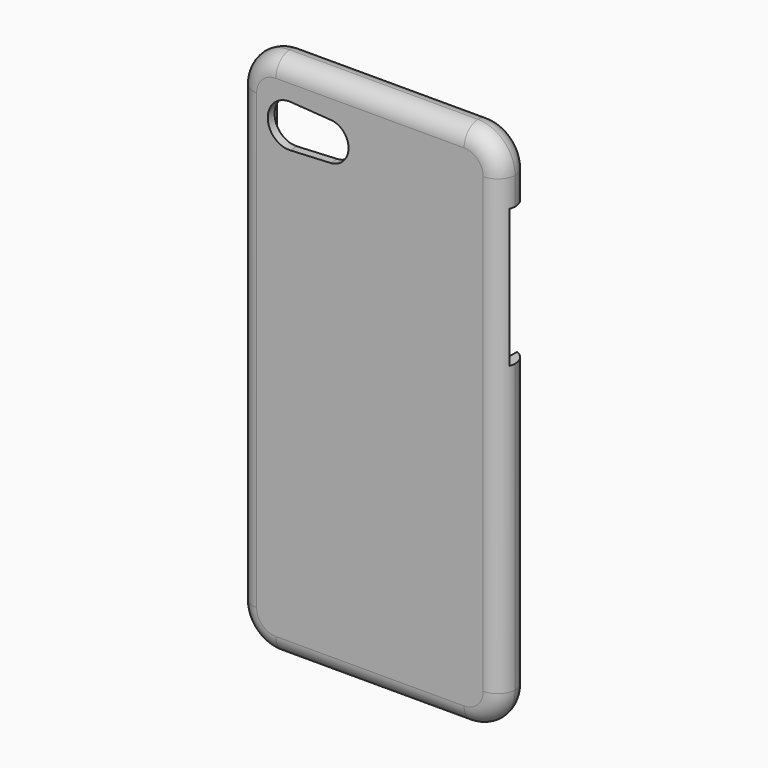
from build123d import *

# Parameters (mm, degrees)
F1_DEPTH      = 9.8298
F2_R          = 10.414
F4_DEPTH      = 7.4422
F6_R          = 10.414
F7_DEPTH      = 25.4
F8_T1_DEPTH   = 126.492
F8_T3_DEPTH   = 52.578
F8_T6_ANGLE   = 90
F8_T8_ANGLE   = 90
F8_T10_ANGLE  = 90
F8_T12_ANGLE  = 90
F9_T1_DEPTH   = 126.492
F9_T3_DEPTH   = 52.578
F9_T6_ANGLE   = 90
F9_T8_ANGLE   = 90
F9_T10_ANGLE  = 90
F9_T12_ANGLE  = 90
F10_W         = 13.4874
F10_H         = 2.8194
F11_DEPTH     = 76.2
F12_W         = 6.6548
F12_H         = 38.608
F13_DEPTH     = 36.7040001
F14_W         = 6.6548
F14_H         = 12.6361389041
F15_DEPTH     = 36.7040001
F16_T1_DEPTH  = 46.228
F16_T6_DEPTH  = 117.348
F16_T11_DEPTH = 117.348
F16_T16_DEPTH = 117.348
F16_T21_ANGLE = 90
F16_T26_ANGLE = 90
F16_T31_ANGLE = 90
F16_T36_ANGLE = 90
F16_T41_DEPTH = 117.348
F16_T46_DEPTH = 117.348
F16_T51_DEPTH = 117.348
F16_T54_ANGLE = 90
F16_T56_ANGLE = 90
F16_T60_DEPTH = 46.228
F16_T66_DEPTH = 46.228
F16_T72_DEPTH = 46.228
F16_T78_DEPTH = 46.228
F16_T83_DEPTH = 46.228


# Not quite as in the source:
# - a fillet or chamfer that OpenCascade refuses, or shapes differently, is made with other operations: its cross-section is extruded or revolved along the edge and cut away or added


with BuildPart() as f1:
    # F0 (on Front) → F1 (new body)
    with BuildSketch(Plane.XZ):
        Polygon((-36.703, -73.66), (36.703, -73.66), (36.703, 73.66), (-26.8460772932, 73.66), (-36.703, 73.66), (-36.703, 59.1852668802), align=None)
        with BuildLine():
            ThreePointArc((-22.2717920435, 52.197646321), (-28.0758079345, 55.8760032584), (-26.5712787061, 62.5807256257))
            ThreePointArc((-26.5712787061, 62.5807256257), (-24.5177487597, 63.7987699714), (-22.1511274544, 64.1145560806))
            Line((-22.1511274544, 64.1145560806), (-10.919338154, 63.3416271462))
            ThreePointArc((-10.919338154, 63.3416271462), (-7.4032650854, 61.6681227759), (-5.9751011246, 58.0454532626))
            ThreePointArc((-5.9751011246, 58.0454532626), (-7.4401434327, 54.3836791207), (-11.0266546305, 52.7429852861))
            Line((-11.0266546305, 52.7429852861), (-22.2717920435, 52.197646321))
        make_face(mode=Mode.SUBTRACT)
    extrude(amount=F1_DEPTH)

    # F2
    f2_edges = [f1.edges().sort_by_distance(p)[0] for p in [
        (36.703, -4.9149, -73.66),
        (36.703, -4.9149, 73.66),
        (-36.703, -4.9149, -73.66),
        (-36.703, -4.9149, 73.66),
    ]]
    fillet(f2_edges, radius=F2_R)

    # F3 (on Front) → F4 (cut)
    with BuildSketch(Plane.XZ):
        Polygon((-33.528, -69.088), (33.528, -69.088), (33.528, 69.088), (-6.3646039926, 69.088), (-33.528, 69.088), (-33.528, -30.0187896937), align=None)
    extrude(amount=F4_DEPTH, mode=Mode.SUBTRACT)

    # F6
    f6_edges = [f1.edges().sort_by_distance(p)[0] for p in [
        (-33.528, -3.7211, 69.088),
        (33.528, -3.7211, 69.088),
        (33.528, -3.7211, -69.088),
        (-33.528, -3.7211, -69.088),
    ]]
    fillet(f6_edges, radius=F6_R)

    # F5 (on Front) → F7 (cut)
    with BuildSketch(Plane.XZ):
        with BuildLine():
            ThreePointArc((17.3579254917, 58.6583771845), (17.3582830329, 58.7237086352), (17.3593556135, 58.7890322592))
            ThreePointArc((17.3593556135, 58.7890322592), (15.6509202483, 62.5470328924), (11.7595014779, 63.924777466))
            ThreePointArc((11.7595014779, 63.924777466), (8.2403525747, 62.2726218117), (6.8081294482, 58.6583771845))
            Line((6.8081294482, 58.6583771845), (17.3579254917, 58.6583771845))
        make_face()
        with BuildLine():
            ThreePointArc((17.3593556135, 58.5277221098), (17.3582830329, 58.5930457338), (17.3579254917, 58.6583771845))
            Line((17.3579254917, 58.6583771845), (6.8081294482, 58.6583771845))
            ThreePointArc((6.8081294482, 58.6583771845), (8.2403525747, 55.0441325573), (11.7595014779, 53.3919769031))
            ThreePointArc((11.7595014779, 53.3919769031), (15.6509202483, 54.7697214767), (17.3593556135, 58.5277221098))
        make_face()
        with BuildLine():
            Line((11.7595014779, 53.3919769031), (22.9592097491, 52.7007143766))
            ThreePointArc((22.9592097491, 52.7007143766), (19.0231520596, 54.5223772758), (17.3593556135, 58.5277221098))
            ThreePointArc((17.3593556135, 58.5277221098), (15.6509202483, 54.7697214767), (11.7595014779, 53.3919769031))
        make_face()
        with BuildLine():
            ThreePointArc((17.3593556135, 58.7890322592), (19.0231520596, 62.7943770932), (22.9592097491, 64.6160399924))
            Line((22.9592097491, 64.6160399924), (11.7595014779, 63.924777466))
            ThreePointArc((11.7595014779, 63.924777466), (15.6509202483, 62.5470328924), (17.3593556135, 58.7890322592))
        make_face()
    extrude(amount=-F7_DEPTH, mode=Mode.SUBTRACT)

    # F8: fillet of radius 5.08 on 1 edges, made by hand

    # F8_s2 → F8_t1 (cut)
    with BuildSketch(Plane.XY.offset(-63.246)):
        with BuildLine():
            ThreePointArc((-31.623, 0), (-35.2151024484, -1.4878975516), (-36.703, -5.08))
            Line((-36.703, -5.08), (-36.703, 0))
            Line((-36.703, 0), (-31.623, 0))
        make_face()
        with BuildLine():
            ThreePointArc((31.623, 0), (35.2151024484, -1.4878975516), (36.703, -5.08))
            Line((36.703, -5.08), (36.703, 0))
            Line((36.703, 0), (31.623, 0))
        make_face()
    extrude(amount=F8_T1_DEPTH, mode=Mode.SUBTRACT)

    # F8_s4 → F8_t3 (cut)
    with BuildSketch(Plane.YZ.offset(-26.289)):
        with BuildLine():
            ThreePointArc((0, -68.58), (-1.4878975516, -72.1721024484), (-5.08, -73.66))
            Line((-5.08, -73.66), (0, -73.66))
            Line((0, -73.66), (0, -68.58))
        make_face()
        with BuildLine():
            ThreePointArc((0, 68.58), (-1.4878975516, 72.1721024484), (-5.08, 73.66))
            Line((-5.08, 73.66), (0, 73.66))
            Line((0, 73.66), (0, 68.58))
        make_face()
    extrude(amount=F8_T3_DEPTH, mode=Mode.SUBTRACT)

    # F8_s5 → F8_t6 (revolve, cut)
    with BuildSketch(Plane.YZ.offset(-26.289)):
        with BuildLine():
            ThreePointArc((0, 68.58), (-1.4878975516, 72.1721024484), (-5.08, 73.66))
            Line((-5.08, 73.66), (0, 73.66))
            Line((0, 73.66), (0, 68.58))
        make_face()
    revolve(axis=Axis((-26.289, 0, 63.246), (0, -1, 0)), revolution_arc=F8_T6_ANGLE, mode=Mode.SUBTRACT)

    # F8_s7 → F8_t8 (revolve, cut)
    with BuildSketch(Plane.YZ.offset(-26.289)):
        with BuildLine():
            ThreePointArc((0, -68.58), (-1.4878975516, -72.1721024484), (-5.08, -73.66))
            Line((-5.08, -73.66), (0, -73.66))
            Line((0, -73.66), (0, -68.58))
        make_face()
    revolve(axis=Axis((-26.289, 0, -63.246), (0, 1, 0)), revolution_arc=F8_T8_ANGLE, mode=Mode.SUBTRACT)

    # F8_s9 → F8_t10 (revolve, cut)
    with BuildSketch(Plane.YZ.offset(26.289)):
        with BuildLine():
            ThreePointArc((0, -68.58), (-1.4878975516, -72.1721024484), (-5.08, -73.66))
            Line((-5.08, -73.66), (0, -73.66))
            Line((0, -73.66), (0, -68.58))
        make_face()
    revolve(axis=Axis((26.289, 0, -63.246), (0, -1, 0)), revolution_arc=F8_T10_ANGLE, mode=Mode.SUBTRACT)

    # F8_s11 → F8_t12 (revolve, cut)
    with BuildSketch(Plane.YZ.offset(26.289)):
        with BuildLine():
            ThreePointArc((0, 68.58), (-1.4878975516, 72.1721024484), (-5.08, 73.66))
            Line((-5.08, 73.66), (0, 73.66))
            Line((0, 73.66), (0, 68.58))
        make_face()
    revolve(axis=Axis((26.289, 0, 63.246), (0, 1, 0)), revolution_arc=F8_T12_ANGLE, mode=Mode.SUBTRACT)

    # F9: fillet of radius 5.08 on 1 edges, made by hand

    # F9_s2 → F9_t1 (cut)
    with BuildSketch(Plane.XY.offset(-63.246)):
        with BuildLine():
            ThreePointArc((-31.6337428592, -9.8298), (-35.1071406193, -8.4568079579), (-36.703, -5.08))
            Line((-36.703, -5.08), (-36.703, -9.8298))
            Line((-36.703, -9.8298), (-31.6337428592, -9.8298))
        make_face()
        with BuildLine():
            ThreePointArc((36.703, -5.08), (35.1071406193, -8.4568079579), (31.6337428592, -9.8298))
            Line((31.6337428592, -9.8298), (36.703, -9.8298))
            Line((36.703, -9.8298), (36.703, -5.08))
        make_face()
    extrude(amount=F9_T1_DEPTH, mode=Mode.SUBTRACT)

    # F9_s4 → F9_t3 (cut)
    with BuildSketch(Plane.YZ.offset(-26.289)):
        with BuildLine():
            ThreePointArc((-9.8298, 68.5907428592), (-8.4568079579, 72.0641406193), (-5.08, 73.66))
            Line((-5.08, 73.66), (-9.8298, 73.66))
            Line((-9.8298, 73.66), (-9.8298, 68.5907428592))
        make_face()
        with BuildLine():
            ThreePointArc((-5.08, -73.66), (-8.4568079579, -72.0641406193), (-9.8298, -68.5907428592))
            Line((-9.8298, -68.5907428592), (-9.8298, -73.66))
            Line((-9.8298, -73.66), (-5.08, -73.66))
        make_face()
    extrude(amount=F9_T3_DEPTH, mode=Mode.SUBTRACT)

    # F9_s5 → F9_t6 (revolve, cut)
    with BuildSketch(Plane.YZ.offset(-26.289)):
        with BuildLine():
            ThreePointArc((-9.8298, -68.5907428592), (-8.4568079579, -72.0641406193), (-5.08, -73.66))
            Line((-5.08, -73.66), (-9.8298, -73.66))
            Line((-9.8298, -73.66), (-9.8298, -68.5907428592))
        make_face()
    revolve(axis=Axis((-26.289, -9.8298, -63.246), (0, 1, 0)), revolution_arc=F9_T6_ANGLE, mode=Mode.SUBTRACT)

    # F9_s7 → F9_t8 (revolve, cut)
    with BuildSketch(Plane.YZ.offset(-26.289)):
        with BuildLine():
            ThreePointArc((-9.8298, 68.5907428592), (-8.4568079579, 72.0641406193), (-5.08, 73.66))
            Line((-5.08, 73.66), (-9.8298, 73.66))
            Line((-9.8298, 73.66), (-9.8298, 68.5907428592))
        make_face()
    revolve(axis=Axis((-26.289, -9.8298, 63.246), (0, -1, 0)), revolution_arc=F9_T8_ANGLE, mode=Mode.SUBTRACT)

    # F9_s9 → F9_t10 (revolve, cut)
    with BuildSketch(Plane.YZ.offset(26.289)):
        with BuildLine():
            ThreePointArc((-9.8298, 68.5907428592), (-8.4568079579, 72.0641406193), (-5.08, 73.66))
            Line((-5.08, 73.66), (-9.8298, 73.66))
            Line((-9.8298, 73.66), (-9.8298, 68.5907428592))
        make_face()
    revolve(axis=Axis((26.289, -9.8298, 63.246), (0, 1, 0)), revolution_arc=F9_T10_ANGLE, mode=Mode.SUBTRACT)

    # F9_s11 → F9_t12 (revolve, cut)
    with BuildSketch(Plane.YZ.offset(26.289)):
        with BuildLine():
            ThreePointArc((-5.08, -73.66), (-8.4568079579, -72.0641406193), (-9.8298, -68.5907428592))
            Line((-9.8298, -68.5907428592), (-9.8298, -73.66))
            Line((-9.8298, -73.66), (-5.08, -73.66))
        make_face()
    revolve(axis=Axis((26.289, -9.8298, -63.246), (0, -1, 0)), revolution_arc=F9_T12_ANGLE, mode=Mode.SUBTRACT)

    # F10 (on Top) → F11 (cut)
    with BuildSketch(Plane.XY):
        Polygon((5.969, -5.0798957236), (5.969, -2.4946516344), (-5.969, -2.4946516344), (-5.969, -6.9396516344), (5.969, -6.9396516344), align=None)
        with Locations((-17.3204755411, -4.7225819435)):
            Rectangle(F10_W, F10_H)
        with Locations((17.3177467659, -4.7195008956)):
            Rectangle(F10_W, F10_H)
    extrude(amount=-F11_DEPTH, mode=Mode.SUBTRACT)

    # F12 (on Right) → F13 (cut, through all)
    with BuildSketch(Plane.YZ):
        with Locations((-3.2993604145, 36.2581742837)):
            Rectangle(F12_W, F12_H)
    extrude(amount=F13_DEPTH, mode=Mode.SUBTRACT)

    # F14 (on Right) → F15 (cut, through all)
    with BuildSketch(Plane.YZ):
        with Locations((-3.3238013398, 35.8446035534)):
            Rectangle(F14_W, F14_H)
    extrude(amount=-F15_DEPTH, mode=Mode.SUBTRACT)

    # F16: fillet of radius 2.54 on 7 edges, made by hand

    # F16_s2 → F16_t1 (join)
    with BuildSketch(Plane.YZ.offset(-23.114)):
        with BuildLine():
            ThreePointArc((-7.4422, 66.548), (-6.6982512242, 68.3440512242), (-4.9022, 69.088))
            Line((-4.9022, 69.088), (-7.4422, 69.088))
            Line((-7.4422, 69.088), (-7.4422, 66.548))
        make_face()
    extrude(amount=F16_T1_DEPTH)


with BuildPart() as f16_tool4:
    # F16_s5 → F16_t6 (new body)
    with BuildSketch(Plane.XY.offset(-58.674)):
        with BuildLine():
            ThreePointArc((-30.988, -7.4422), (-32.7840512242, -6.6982512242), (-33.528, -4.9022))
            Line((-33.528, -4.9022), (-33.528, -7.4422))
            Line((-33.528, -7.4422), (-30.988, -7.4422))
        make_face()
    extrude(amount=F16_T6_DEPTH)

    split(bisect_by=Plane.XZ.offset(6.6512013398), keep=Keep.TOP)


with BuildPart() as f1_1:
    add(f1.part)

    # F16_t3: union F16_tool4
    add(f16_tool4.part)


with BuildPart() as f16_tool9:
    # F16_s10 → F16_t11 (new body)
    with BuildSketch(Plane.XY.offset(-58.674)):
        with BuildLine():
            ThreePointArc((-30.988, -7.4422), (-32.7840512242, -6.6982512242), (-33.528, -4.9022))
            Line((-33.528, -4.9022), (-33.528, -7.4422))
            Line((-33.528, -7.4422), (-30.988, -7.4422))
        make_face()
    extrude(amount=F16_T11_DEPTH)

    split(bisect_by=Plane.XY.offset(29.5265341014), keep=Keep.BOTTOM)


with BuildPart() as f1_2:
    add(f1_1.part)

    # F16_t8: union F16_tool9
    add(f16_tool9.part)


with BuildPart() as f16_tool14:
    # F16_s15 → F16_t16 (new body)
    with BuildSketch(Plane.XY.offset(-58.674)):
        with BuildLine():
            ThreePointArc((-30.988, -7.4422), (-32.7840512242, -6.6982512242), (-33.528, -4.9022))
            Line((-33.528, -4.9022), (-33.528, -7.4422))
            Line((-33.528, -7.4422), (-30.988, -7.4422))
        make_face()
    extrude(amount=F16_T16_DEPTH)

    split(bisect_by=Plane.XY.offset(42.1626730055), keep=Keep.TOP)


with BuildPart() as f1_3:
    add(f1_2.part)

    # F16_t13: union F16_tool14
    add(f16_tool14.part)


with BuildPart() as f16_tool19:
    # F16_s20 → F16_t21 (revolve)
    with BuildSketch(Plane.YZ.offset(23.114)):
        with BuildLine():
            ThreePointArc((-4.9022, -69.088), (-6.6982512242, -68.3440512242), (-7.4422, -66.548))
            Line((-7.4422, -66.548), (-7.4422, -69.088))
            Line((-7.4422, -69.088), (-4.9022, -69.088))
        make_face()
    revolve(axis=Axis((23.114, -7.4422, -58.674), (0, -1, 0)), revolution_arc=F16_T21_ANGLE)

    split(bisect_by=Plane.XZ.offset(6.1292008956), keep=Keep.TOP)


with BuildPart() as f1_4:
    add(f1_3.part)

    # F16_t18: union F16_tool19
    add(f16_tool19.part)


with BuildPart() as f16_tool24:
    # F16_s25 → F16_t26 (revolve)
    with BuildSketch(Plane.YZ.offset(23.114)):
        with BuildLine():
            ThreePointArc((-4.9022, -69.088), (-6.6982512242, -68.3440512242), (-7.4422, -66.548))
            Line((-7.4422, -66.548), (-7.4422, -69.088))
            Line((-7.4422, -69.088), (-4.9022, -69.088))
        make_face()
    revolve(axis=Axis((23.114, -7.4422, -58.674), (0, -1, 0)), revolution_arc=F16_T26_ANGLE)

    split(bisect_by=Plane.YZ.offset(24.0614467659), keep=Keep.TOP)


with BuildPart() as f1_5:
    add(f1_4.part)

    # F16_t23: union F16_tool24
    add(f16_tool24.part)


with BuildPart() as f16_tool29:
    # F16_s30 → F16_t31 (revolve)
    with BuildSketch(Plane.YZ.offset(-23.114)):
        with BuildLine():
            ThreePointArc((-7.4422, -66.548), (-6.6982512242, -68.3440512242), (-4.9022, -69.088))
            Line((-4.9022, -69.088), (-7.4422, -69.088))
            Line((-7.4422, -69.088), (-7.4422, -66.548))
        make_face()
    revolve(axis=Axis((-23.114, -7.4422, -58.674), (0, 1, 0)), revolution_arc=F16_T31_ANGLE)

    split(bisect_by=Plane.XZ.offset(6.1322819435), keep=Keep.TOP)


with BuildPart() as f1_6:
    add(f1_5.part)

    # F16_t28: union F16_tool29
    add(f16_tool29.part)


with BuildPart() as f16_tool34:
    # F16_s35 → F16_t36 (revolve)
    with BuildSketch(Plane.YZ.offset(-23.114)):
        with BuildLine():
            ThreePointArc((-7.4422, -66.548), (-6.6982512242, -68.3440512242), (-4.9022, -69.088))
            Line((-4.9022, -69.088), (-7.4422, -69.088))
            Line((-7.4422, -69.088), (-7.4422, -66.548))
        make_face()
    revolve(axis=Axis((-23.114, -7.4422, -58.674), (0, 1, 0)), revolution_arc=F16_T36_ANGLE)

    split(bisect_by=Plane.YZ.offset(-24.0641755411), keep=Keep.BOTTOM)


with BuildPart() as f1_7:
    add(f1_6.part)

    # F16_t33: union F16_tool34
    add(f16_tool34.part)


with BuildPart() as f16_tool39:
    # F16_s40 → F16_t41 (new body)
    with BuildSketch(Plane.XY.offset(-58.674)):
        with BuildLine():
            ThreePointArc((30.988, -7.4422), (32.7840512242, -6.6982512242), (33.528, -4.9022))
            Line((33.528, -4.9022), (33.528, -7.4422))
            Line((33.528, -7.4422), (30.988, -7.4422))
        make_face()
    extrude(amount=F16_T41_DEPTH)

    split(bisect_by=Plane.XZ.offset(6.6267604145), keep=Keep.TOP)


with BuildPart() as f1_8:
    add(f1_7.part)

    # F16_t38: union F16_tool39
    add(f16_tool39.part)


with BuildPart() as f16_tool44:
    # F16_s45 → F16_t46 (new body)
    with BuildSketch(Plane.XY.offset(-58.674)):
        with BuildLine():
            ThreePointArc((30.988, -7.4422), (32.7840512242, -6.6982512242), (33.528, -4.9022))
            Line((33.528, -4.9022), (33.528, -7.4422))
            Line((33.528, -7.4422), (30.988, -7.4422))
        make_face()
    extrude(amount=F16_T46_DEPTH)

    split(bisect_by=Plane.XY.offset(16.9541742837), keep=Keep.BOTTOM)


with BuildPart() as f1_9:
    add(f1_8.part)

    # F16_t43: union F16_tool44
    add(f16_tool44.part)


with BuildPart() as f16_tool49:
    # F16_s50 → F16_t51 (new body)
    with BuildSketch(Plane.XY.offset(-58.674)):
        with BuildLine():
            ThreePointArc((30.988, -7.4422), (32.7840512242, -6.6982512242), (33.528, -4.9022))
            Line((33.528, -4.9022), (33.528, -7.4422))
            Line((33.528, -7.4422), (30.988, -7.4422))
        make_face()
    extrude(amount=F16_T51_DEPTH)

    split(bisect_by=Plane.XY.offset(55.5621742837), keep=Keep.TOP)


with BuildPart() as f1_10:
    add(f1_9.part)

    # F16_t48: union F16_tool49
    add(f16_tool49.part)

    # F16_s53 → F16_t54 (revolve)
    with BuildSketch(Plane.YZ.offset(-23.114)):
        with BuildLine():
            ThreePointArc((-7.4422, 66.548), (-6.6982512242, 68.3440512242), (-4.9022, 69.088))
            Line((-4.9022, 69.088), (-7.4422, 69.088))
            Line((-7.4422, 69.088), (-7.4422, 66.548))
        make_face()
    revolve(axis=Axis((-23.114, -7.4422, 58.674), (0, -1, 0)), revolution_arc=F16_T54_ANGLE)

    # F16_s55 → F16_t56 (revolve)
    with BuildSketch(Plane.XY.offset(58.674)):
        with BuildLine():
            ThreePointArc((30.988, -7.4422), (32.7840512242, -6.6982512242), (33.528, -4.9022))
            Line((33.528, -4.9022), (33.528, -7.4422))
            Line((33.528, -7.4422), (30.988, -7.4422))
        make_face()
    revolve(axis=Axis((23.114, -7.4422, 58.674), (0, -1, 0)), revolution_arc=F16_T56_ANGLE)


with BuildPart() as f16_tool58:
    # F16_s59 → F16_t60 (new body)
    with BuildSketch(Plane.YZ.offset(-23.114)):
        with BuildLine():
            ThreePointArc((-4.9022, -69.088), (-6.6982512242, -68.3440512242), (-7.4422, -66.548))
            Line((-7.4422, -66.548), (-7.4422, -69.088))
            Line((-7.4422, -69.088), (-4.9022, -69.088))
        make_face()
    extrude(amount=F16_T60_DEPTH)

    split(bisect_by=Plane.YZ.offset(-10.5767755411), keep=Keep.TOP)

    split(bisect_by=Plane.YZ.offset(-5.969), keep=Keep.BOTTOM)


with BuildPart() as f1_11:
    add(f1_10.part)

    # F16_t57: union F16_tool58
    add(f16_tool58.part)


with BuildPart() as f16_tool64:
    # F16_s65 → F16_t66 (new body)
    with BuildSketch(Plane.YZ.offset(-23.114)):
        with BuildLine():
            ThreePointArc((-4.9022, -69.088), (-6.6982512242, -68.3440512242), (-7.4422, -66.548))
            Line((-7.4422, -66.548), (-7.4422, -69.088))
            Line((-7.4422, -69.088), (-4.9022, -69.088))
        make_face()
    extrude(amount=F16_T66_DEPTH)

    split(bisect_by=Plane.XZ.offset(6.1322819435), keep=Keep.TOP)

    split(bisect_by=Plane.YZ.offset(-5.969), keep=Keep.BOTTOM)


with BuildPart() as f1_12:
    add(f1_11.part)

    # F16_t63: union F16_tool64
    add(f16_tool64.part)


with BuildPart() as f16_tool70:
    # F16_s71 → F16_t72 (new body)
    with BuildSketch(Plane.YZ.offset(-23.114)):
        with BuildLine():
            ThreePointArc((-4.9022, -69.088), (-6.6982512242, -68.3440512242), (-7.4422, -66.548))
            Line((-7.4422, -66.548), (-7.4422, -69.088))
            Line((-7.4422, -69.088), (-4.9022, -69.088))
        make_face()
    extrude(amount=F16_T72_DEPTH)

    split(bisect_by=Plane.YZ.offset(10.5740467659), keep=Keep.BOTTOM)

    split(bisect_by=Plane.YZ.offset(5.969), keep=Keep.TOP)


with BuildPart() as f1_13:
    add(f1_12.part)

    # F16_t69: union F16_tool70
    add(f16_tool70.part)


with BuildPart() as f16_tool76:
    # F16_s77 → F16_t78 (new body)
    with BuildSketch(Plane.YZ.offset(-23.114)):
        with BuildLine():
            ThreePointArc((-4.9022, -69.088), (-6.6982512242, -68.3440512242), (-7.4422, -66.548))
            Line((-7.4422, -66.548), (-7.4422, -69.088))
            Line((-7.4422, -69.088), (-4.9022, -69.088))
        make_face()
    extrude(amount=F16_T78_DEPTH)

    split(bisect_by=Plane.XZ.offset(6.9396516344), keep=Keep.TOP)


with BuildPart() as f1_14:
    add(f1_13.part)

    # F16_t75: union F16_tool76
    add(f16_tool76.part)


with BuildPart() as f16_tool81:
    # F16_s82 → F16_t83 (new body)
    with BuildSketch(Plane.YZ.offset(-23.114)):
        with BuildLine():
            ThreePointArc((-4.9022, -69.088), (-6.6982512242, -68.3440512242), (-7.4422, -66.548))
            Line((-7.4422, -66.548), (-7.4422, -69.088))
            Line((-7.4422, -69.088), (-4.9022, -69.088))
        make_face()
    extrude(amount=F16_T83_DEPTH)

    split(bisect_by=Plane.XZ.offset(6.1292008956), keep=Keep.TOP)

    split(bisect_by=Plane.YZ.offset(5.969), keep=Keep.TOP)


with BuildPart() as f1_15:
    add(f1_14.part)

    # F16_t80: union F16_tool81
    add(f16_tool81.part)


solid = f1_15.part
